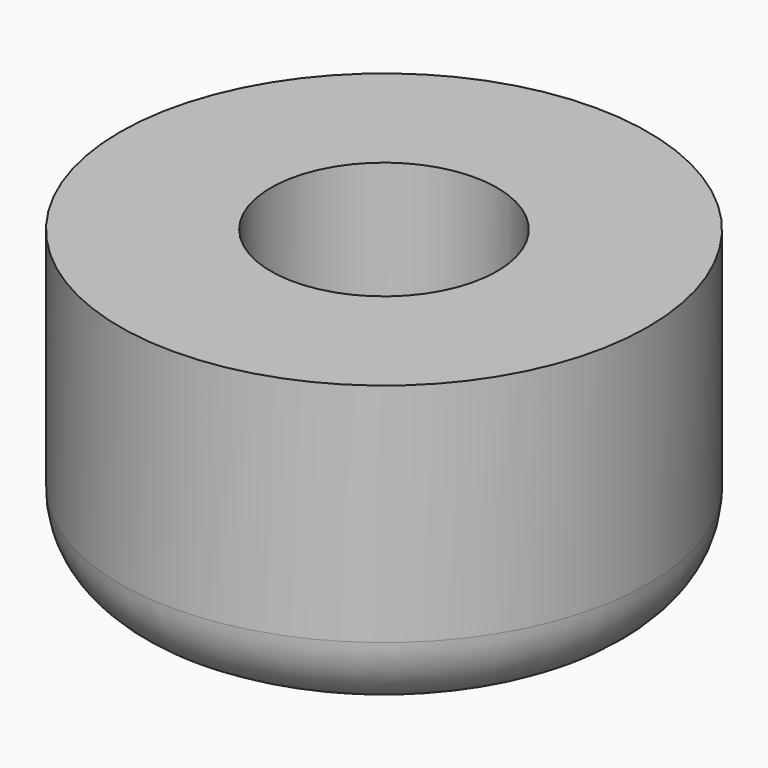
from build123d import *

# Parameters (mm, degrees)
F0_R     = 3.5
F0_R_2   = 1.5
F1_DEPTH = 3
F2_R     = 3.5
F3_DEPTH = 1
F4_R     = 0.99999


# Not quite as in the source:
# - a fillet or chamfer is up to 0.001 mm smaller than in the source, because OpenCascade refuses the exact size


with BuildPart() as f1:
    # F0 (on Top) → F1 (new body)
    with BuildSketch(Plane.XY):
        Circle(F0_R)
        Circle(F0_R_2, mode=Mode.SUBTRACT)
    extrude(amount=F1_DEPTH)

    # F2 (on Top) → F3 (join)
    with BuildSketch(Plane.XY):
        Circle(F2_R)
    extrude(amount=-F3_DEPTH)

    # F4 (radius 1 in the source; OpenCascade refuses exactly that, so slightly less here)
    f4_edges = [f1.edges().sort_by_distance(p)[0] for p in [
        (-3.5, 0, -1),
    ]]
    fillet(f4_edges, radius=F4_R)


solid = f1.part
